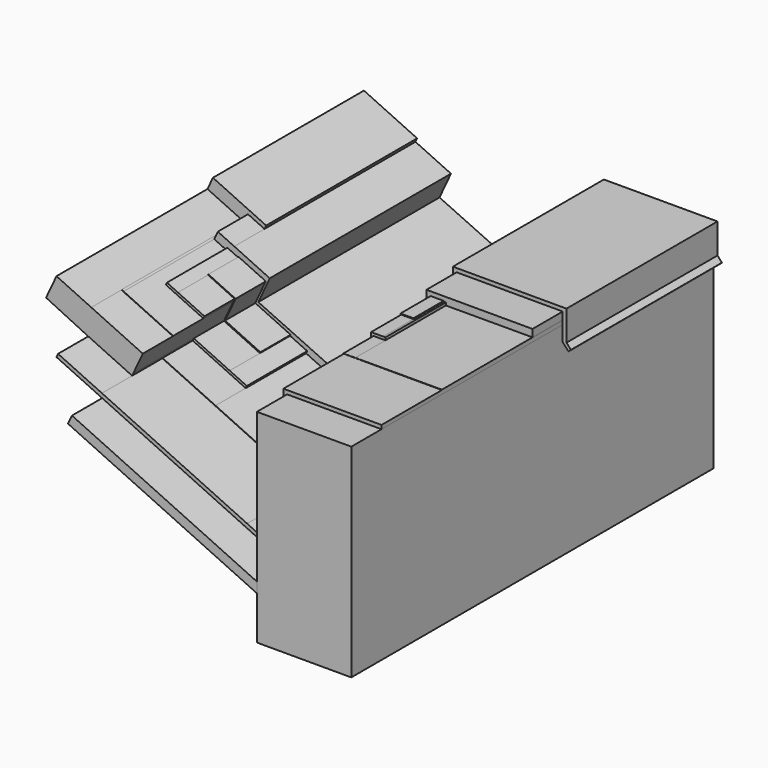
from build123d import *

# Parameters (mm, degrees)
F1_DEPTH  = 120
F2_DEPTH  = 120
F3_DEPTH  = 110
F4_DEPTH  = 100
F5_DEPTH  = 100
F6_DEPTH  = 90
F7_DEPTH  = 90
F8_DEPTH  = 80
F9_DEPTH  = 80
F10_DEPTH = 80
F11_DEPTH = 80
F12_DEPTH = 70
F13_DEPTH = 70
F14_DEPTH = 70
F15_DEPTH = 60
F16_DEPTH = 50
F17_DEPTH = 50


with BuildPart() as f1:
    # F0 (on Front) → F1 (new body)
    with BuildSketch(Plane.XZ):
        Polygon((62.7532724798, 38.0357114375), (37.7532724798, 38.0357114375), (37.7532724798, -1.5682141957), (37.7532724798, -4.3017355892), (37.7532724798, -15.7766969041), (62.7532724798, -15.7766969041), (62.7532724798, 33.9487026308), align=None)
    extrude(amount=F1_DEPTH)


with BuildPart() as f2:
    # F0 (on Front) → F2 (new body)
    with BuildSketch(Plane.XZ):
        Polygon((37.7532724798, -4.3017355892), (37.7532724798, -1.5682141957), (-11.2419818741, 21.2279597301), (-12.2874860827, 18.9808833218), align=None)
    extrude(amount=F2_DEPTH)


with BuildPart() as f3:
    # F0 (on Front) → F3 (new body)
    with BuildSketch(Plane.XZ):
        Polygon((37.7532724798, -1.5682141957), (37.7532724798, 38.0357114375), (62.7532724798, 38.0357114375), (62.7532724798, 39.0357114375), (36.7532724798, 39.0357114375), (36.7532724798, 9.1857140462), (36.7532724798, 0), (27.1622682206, 4.462436293), (-11.3030609789, 22.3593192893), (-22.9213011947, 27.7649739423), (-23.3431488375, 26.8583072085), (-11.2419818741, 21.2279597301), align=None)
    extrude(amount=F3_DEPTH)


with BuildPart() as f4:
    # F0 (on Front) → F4 (new body)
    with BuildSketch(Plane.XZ):
        Polygon((-34.093962769, 33.1498159787), (-22.9213011947, 27.7649739423), (-11.3030609789, 22.3593192893), (-11.2608762147, 22.4499859627), (-10.978238294, 23.0574526744), (-8.4797753205, 28.427337519), (-22.130522729, 34.7786630963), (-31.3420099408, 39.0645203158), align=None)
    extrude(amount=F4_DEPTH)


with BuildPart() as f5:
    # F0 (on Front) → F5 (new body)
    with BuildSketch(Plane.XZ):
        Polygon((36.7532724798, 0), (36.7532724798, 9.1857140462), (27.1622682206, 4.462436293), align=None)
    extrude(amount=F5_DEPTH)


with BuildPart() as f6:
    # F0 (on Front) → F6 (new body)
    with BuildSketch(Plane.XZ):
        Polygon((-22.0883379648, 34.8693297696), (-22.130522729, 34.7786630963), (-8.4797753205, 28.427337519), (-8.4375905562, 28.5180041924), (-18.3633532114, 33.1361945624), (-21.5590084305, 34.6230469758), align=None)
    extrude(amount=F6_DEPTH)


with BuildPart() as f7:
    # F0 (on Front) → F7 (new body)
    with BuildSketch(Plane.XZ):
        Polygon((36.7532724798, 39.0357114375), (62.7532724798, 39.0357114375), (62.7528878644, 39.1357106978), (39.7976157027, 39.102147702), (36.6532724798, 39.0975503451), (36.6532724798, 36.1267757076), (36.6532724798, 15.0731514328), (36.6532724798, 9.2479357519), (27.1610418439, 4.5733010026), (20.5657351541, 7.641919798), (2.7888639591, 15.9130197843), (-11.2608762147, 22.4499859627), (-11.3030609789, 22.3593192893), (27.1622682206, 4.462436293), (36.7532724798, 9.1857140462), align=None)
    extrude(amount=F7_DEPTH)


with BuildPart() as f8:
    # F0 (on Front) → F8 (new body)
    with BuildSketch(Plane.XZ):
        Polygon((-18.3633532114, 33.1361945624), (-8.4375905562, 28.5180041924), (-8.1549526356, 29.1254709041), (-15.182753971, 32.3953178244), (-18.0807152907, 33.743661274), align=None)
    extrude(amount=F8_DEPTH)


with BuildPart() as f9:
    # F0 (on Front) → F9 (new body)
    with BuildSketch(Plane.XZ):
        Polygon((-10.978238294, 23.0574526744), (-11.2608762147, 22.4499859627), (2.7888639591, 15.9130197843), (3.0715018798, 16.520486496), (-1.4491225172, 18.6238114275), align=None)
    extrude(amount=F9_DEPTH)


with BuildPart() as f10:
    # F0 (on Front) → F10 (new body)
    with BuildSketch(Plane.XZ):
        Polygon((36.6532724798, 9.2479357519), (36.6532724798, 15.0731514328), (35.6532724798, 15.0731514328), (35.6532724798, 13.1126534771), (35.6532724798, 9.8701528088), (27.1487780767, 5.6819480983), (22.5392122094, 7.8266551035), (22.3868255866, 7.8975565001), (20.9875827969, 8.5485865318), (20.5657351541, 7.641919798), (27.1610418439, 4.5733010026), align=None)
    extrude(amount=F10_DEPTH)


with BuildPart() as f11:
    # F0 (on Front) → F11 (new body)
    with BuildSketch(Plane.XZ):
        Polygon((36.6532724798, 39.0975503451), (39.7976157027, 39.102147702), (39.793651551, 39.8057106978), (39.2196251732, 39.8024764065), (35.9832724798, 39.7842415175), (35.9832724798, 36.6213790533), (35.9832724798, 36.1267757076), (36.6532724798, 36.1267757076), align=None)
    extrude(amount=F11_DEPTH)


with BuildPart() as f12:
    # F0 (on Front) → F12 (new body)
    with BuildSketch(Plane.XZ):
        Polygon((-8.4797753205, 28.427337519), (-10.978238294, 23.0574526744), (-1.4491225172, 18.6238114275), (-1.3221520646, 18.8967058894), (-10.6699344947, 23.2459776078), (-7.8892497602, 29.2224347223), (-15.0983844425, 32.5766511712), (-15.182753971, 32.3953178244), (-8.1549526356, 29.1254709041), (-8.4375905562, 28.5180041924), align=None)
    extrude(amount=F12_DEPTH)


with BuildPart() as f13:
    # F0 (on Front) → F13 (new body)
    with BuildSketch(Plane.XZ):
        Polygon((35.6532724798, 9.8701528088), (35.6532724798, 13.1126534771), (35.4532724798, 13.1126534771), (35.4532724798, 9.9945962201), (27.1500502265, 5.9019444202), (22.623581738, 8.0079884503), (22.5392122094, 7.8266551035), (27.1487780767, 5.6819480983), align=None)
    extrude(amount=F13_DEPTH)


with BuildPart() as f14:
    # F0 (on Front) → F14 (new body)
    with BuildSketch(Plane.XZ):
        Polygon((35.9832724798, 39.7842415175), (39.2196251732, 39.8024764065), (39.2196251732, 40.0024764065), (35.7832724798, 40.0024764065), (35.7832724798, 36.6213790533), (35.9832724798, 36.6213790533), align=None)
    extrude(amount=F14_DEPTH)


with BuildPart() as f15:
    # F0 (on Front) → F15 (new body)
    with BuildSketch(Plane.XZ):
        Polygon((39.7976157027, 39.102147702), (62.7528878644, 39.1357106978), (62.7532724798, 41.0975503451), (47.1063793285, 41.0975503451), (46.2950781567, 41.0975503451), (34.6532724798, 41.0975503451), (34.6532724798, 33.1212431192), (34.6532724798, 16.1968208849), (33.6532724798, 13.4902799919), (33.6532724798, 11.3371306487), (27.2846735988, 8.1965293971), (23.4195049673, 9.6229607518), (20.8119284672, 9.6229607518), (-9.8889558036, 23.7389743125), (-6.8471991162, 30.2765469362), (-16.2509841568, 34.6518751628), (-20.6033906013, 36.6769328059), (-21.5590084305, 34.6230469758), (-18.3633532114, 33.1361945624), (-18.0807152907, 33.743661274), (-15.182753971, 32.3953178244), (-15.0983844425, 32.5766511712), (-7.8892497602, 29.2224347223), (-10.6699344947, 23.2459776078), (-1.3221520646, 18.8967058894), (-1.4491225172, 18.6238114275), (3.0715018798, 16.520486496), (2.7888639591, 15.9130197843), (20.5657351541, 7.641919798), (20.9875827969, 8.5485865318), (22.3868255866, 7.8975565001), (22.5392122094, 7.8266551035), (22.623581738, 8.0079884503), (27.1500502265, 5.9019444202), (35.4532724798, 9.9945962201), (35.4532724798, 13.1126534771), (35.6532724798, 13.1126534771), (35.6532724798, 15.0731514328), (36.6532724798, 15.0731514328), (36.6532724798, 36.1267757076), (35.9832724798, 36.1267757076), (35.9832724798, 36.6213790533), (35.7832724798, 36.6213790533), (35.7832724798, 40.0024764065), (39.2196251732, 40.0024764065), (39.2196251732, 39.8024764065), (39.793651551, 39.8057106978), align=None)
    extrude(amount=F15_DEPTH)


with BuildPart() as f16:
    # F0 (on Front) → F16 (new body)
    with BuildSketch(Plane.XZ):
        Polygon((-29.9015114106, 42.1605482769), (-31.3420099408, 39.0645203158), (-22.130522729, 34.7786630963), (-22.0883379648, 34.8693297696), (-21.5590084305, 34.6230469758), (-20.6033906013, 36.6769328059), (-16.2509841568, 34.6518751628), (-15.8082882201, 35.6033506205), align=None)
    extrude(amount=F16_DEPTH)


with BuildPart() as f17:
    # F0 (on Front) → F17 (new body)
    with BuildSketch(Plane.XZ):
        Polygon((62.7532724798, 39.0357114375), (62.7532724798, 38.0357114375), (62.7532724798, 33.9487026308), (64.2652862209, 32.2687230941), (64.9227538708, 32.8604565643), (63.7534983963, 34.1596016824), (63.7534983963, 42.0975503451), (33.6532724798, 42.0975503451), (33.6532724798, 33.7673542435), (32.3305874402, 33.1794772946), (32.7367356742, 32.2656700874), (34.6532724798, 33.1212431192), (34.6532724798, 41.0975503451), (46.2950781567, 41.0975503451), (47.1063793285, 41.0975503451), (62.7532724798, 41.0975503451), (62.7528878644, 39.1357106978), align=None)
    extrude(amount=F17_DEPTH)


solid = Compound([f1.part, f2.part, f3.part, f4.part, f5.part, f6.part, f7.part, f8.part, f9.part, f10.part, f11.part, f12.part, f13.part, f14.part, f15.part, f16.part, f17.part])
